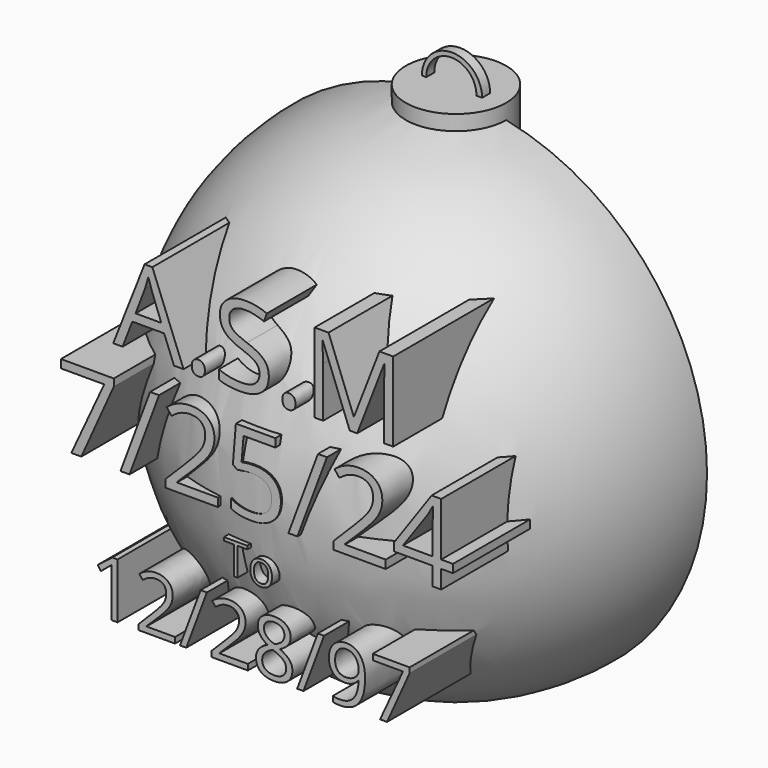
from build123d import *

# Parameters (mm, degrees)
F1_ANGLE       = 180
F2_TEXT_SIZE   = 14.0563843565
F2_TEXT_SIZE_2 = 5.5695107828
F2_TEXT_SIZE_3 = 9.8127988167
F3_DEPTH       = 31.75
F4_R           = 6.35
F5_DEPTH       = 33.02
F7_DEPTH       = 0.635
F9_DEPTH       = 6.3510001
F10_DEPTH      = 25.4


# Not quite as in the source:
# - Text() gives the source's letters only with a copy of the font that has no kerning and outlines rounded to 1/6400 em; it was checked with that copy


with BuildPart() as f1:
    # F0 (on Front) → F1 (revolve)
    with BuildSketch(Plane.XZ):
        with BuildLine():
            ThreePointArc((-31.75, 0), (0, -31.75), (31.75, 0))
            Line((31.75, 0), (-31.75, 0))
        make_face()
    revolve(axis=Axis((0, 0, 0), (-1, 0, 0)), revolution_arc=F1_ANGLE)

    # F2 (on Front) → F3 (join)
    with BuildSketch(Plane.XZ):
        with Locations((-17.9497376084, 11.2663246691)):
            Text('A.S.M', F2_TEXT_SIZE, font='Open Sans', text_align=(TextAlign.LEFT, TextAlign.BOTTOM))
        with Locations((-25.2060100902, -2.6733647101)):
            Text('7/25/24', F2_TEXT_SIZE, font='Open Sans', text_align=(TextAlign.LEFT, TextAlign.BOTTOM))
        with Locations((-4.0100479964, -9.7386874259)):
            Text('To', F2_TEXT_SIZE_2, font='Open Sans', text_align=(TextAlign.LEFT, TextAlign.BOTTOM))
        with Locations((-20.8274237812, -19.636310637)):
            Text('12/28/97', F2_TEXT_SIZE_3, font='Open Sans', text_align=(TextAlign.LEFT, TextAlign.BOTTOM))
    extrude(amount=F3_DEPTH)

    # F4 (on Top) → F5 (join)
    with BuildSketch(Plane.XY):
        Circle(F4_R)
    extrude(amount=F5_DEPTH)

    # F6 (on Front) → F7 (join, symmetric)
    with BuildSketch(Plane.XZ):
        with BuildLine():
            ThreePointArc((3.81, 33.02), (0, 36.83), (-3.81, 33.02))
            Line((-3.81, 33.02), (3.81, 33.02))
        make_face()
    extrude(amount=F7_DEPTH, both=True)

    # F8 (on Front) → F9 (cut, through all)
    with BuildSketch(Plane.XZ):
        with BuildLine():
            ThreePointArc((3.094369136, 33.02), (-0.0802359729, 36.2450739717), (-3.2548410818, 33.02))
            Line((-3.2548410818, 33.02), (3.094369136, 33.02))
        make_face()
    extrude(amount=-F9_DEPTH, mode=Mode.SUBTRACT)

    # F8 (on Front) → F10 (cut)
    with BuildSketch(Plane.XZ):
        with BuildLine():
            ThreePointArc((3.094369136, 33.02), (-0.0802359729, 36.2450739717), (-3.2548410818, 33.02))
            Line((-3.2548410818, 33.02), (3.094369136, 33.02))
        make_face()
    extrude(amount=F10_DEPTH, mode=Mode.SUBTRACT)


solid = f1.part
